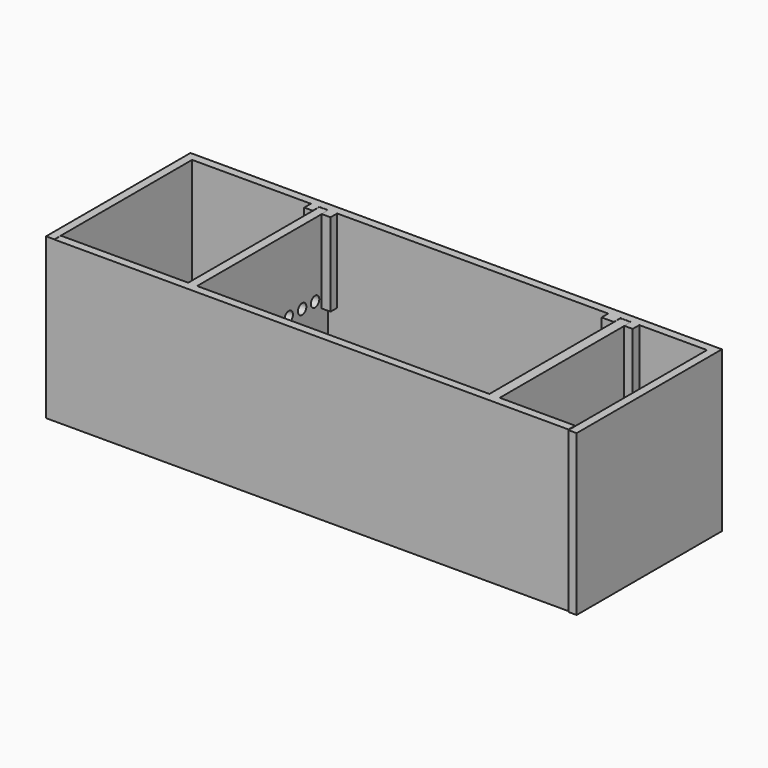
from build123d import *

# Parameters (mm, degrees)
F0_W      = 124.1378337145
F0_H      = 39.50663656
F1_DEPTH  = 3
F2_W      = 2.5017783046
F2_H      = 39.50663656
F2_W_2    = 2.1480806172
F3_DEPTH  = 17.78
F5_DEPTH  = 17.78
F7_D      = 2.54
F8_W      = 30.6726247072
F8_H      = 35.56
F8_W_2    = 18.1720815599
F8_W_3    = 70.4594738781
F9_DEPTH  = 2
F11_DEPTH = 2
F13_DEPTH = 2
F15_DEPTH = 2
F16_W     = 2.9533728957
F16_H     = 20.0437232852
F16_W_2   = 2.1480806172
F16_H_2   = 20.0032039857
F16_W_3   = 2.0457915962
F17_DEPTH = 2


with BuildPart() as f1:
    # F0 (on Top) → F1 (new body)
    with BuildSketch(Plane.XY):
        Rectangle(F0_W, F0_H)
    extrude(amount=F1_DEPTH)

    # F2 (on face) → F3 (join)
    with BuildSketch(Plane.XY.offset(3)):
        with Locations((42.4621514976, 0)):
            Rectangle(F2_W, F2_H)
        with Locations((-30.3222518414, 0)):
            Rectangle(F2_W_2, F2_H)
    extrude(amount=F3_DEPTH)

    # F5 (add): faces of the model
    f5_faces = [f1.faces().sort_by_distance(p)[0] for p in [
        (-30.3222518414, 0, 20.78),
        (42.4621514976, 0, 20.78),
    ]]
    extrude(f5_faces, amount=F5_DEPTH)

    # F7 (through all)
    with Locations(Plane(origin=(-31.39629215, 0, 0), x_dir=(0, -1, 0), z_dir=(-1, 0, 0))):
        with Locations((-11.8883280084, 20.8021104336), (-15.7889463007, 20.7917392254), (-7.8511117026, 20.7805093378), (-3.6703720689, 20.7868441939)):
            Hole(F7_D / 2)

    # F8 (on face) → F9 (join)
    with BuildSketch(Plane.XZ.offset(19.75331828)):
        Polygon((-62.0689168572, 3), (-62.0689168572, 0), (61.8851222098, 0), (61.8851222098, 3), (43.7130406499, 3), (43.7130406499, 38.56), (41.2112623453, 38.56), (41.2112623453, 3), (-29.2482115328, 3), (-29.2482115328, 38.56), (-31.39629215, 38.56), (-31.39629215, 3), align=None)
        with Locations((-46.7326045036, 20.78)):
            Rectangle(F8_W, F8_H)
        with Locations((52.7990814298, 20.78)):
            Rectangle(F8_W_2, F8_H)
        with Locations((5.9815254062, 20.78)):
            Rectangle(F8_W_3, F8_H)
    extrude(amount=F9_DEPTH)

    # F10 (on face) → F11 (join)
    with BuildSketch(Plane(origin=(0, 19.75331828, 0), x_dir=(-1, 0, 0), z_dir=(0, 1, 0))):
        Polygon((-62.0689168572, 38.6005192995), (-62.0689168572, 3), (-43.7130406499, 3), (-43.7130406499, 38.56), (-41.2112623453, 38.56), (-41.2112623453, 3), (29.2482115328, 3), (29.2482115328, 38.56), (31.39629215, 38.56), (31.39629215, 3), (62.0689168572, 3), (62.0689168572, 38.6005192995), align=None)
        Polygon((-62.0689168572, 3), (-62.0689168572, 0), (62.0689168572, 0), (62.0689168572, 3), (31.39629215, 3), (31.39629215, 38.56), (29.2482115328, 38.56), (29.2482115328, 3), (-41.2112623453, 3), (-41.2112623453, 38.56), (-43.7130406499, 38.56), (-43.7130406499, 3), align=None)
    extrude(amount=F11_DEPTH)

    # F12 (on face) → F13 (join)
    with BuildSketch(Plane.YZ.offset(62.0689168572)):
        Polygon((19.75331828, 3), (19.75331828, 38.6005192995), (-22.0371708274, 38.6005192995), (-22.0371708274, 0), (-19.75331828, 0), (-19.75331828, 3), align=None)
        Polygon((21.75331828, 0), (21.75331828, 38.6005192995), (19.75331828, 38.6005192995), (19.75331828, 3), (-19.75331828, 3), (-19.75331828, 0), align=None)
    extrude(amount=F13_DEPTH)

    # F14 (on face) → F15 (join)
    with BuildSketch(Plane(origin=(-62.0689168572, 0, 0), x_dir=(0, -1, 0), z_dir=(-1, 0, 0))):
        Polygon((-21.75331828, 0), (21.75331828, 0), (21.75331828, 38.56), (19.75331828, 38.56), (19.75331828, 3), (-19.75331828, 3), (-19.75331828, 38.6005192995), (-21.75331828, 38.6005192995), align=None)
        Polygon((19.75331828, 38.56), (21.75331828, 38.56), (21.75331828, 38.6005192995), (-19.75331828, 38.6005192995), (-19.75331828, 3), (19.75331828, 3), align=None)
    extrude(amount=F15_DEPTH)

    # F16 (on face) → F17 (join)
    with BuildSketch(Plane.XZ.offset(-19.75331828)):
        with Locations((39.7345758975, 28.5786576569)):
            Rectangle(F16_W, F16_H)
        with Locations((-30.3222518414, 28.5583980072)):
            Rectangle(F16_W_2, F16_H_2)
        Polygon((-33.4356613457, 18.5567960143), (-31.39629215, 18.5567960143), (-31.39629215, 38.56), (-31.39629215, 38.6005192995), (-33.4356613457, 38.6005192995), align=None)
        Polygon((-29.2482115328, 38.56), (-29.2482115328, 18.5567960143), (-27.0928554237, 18.5567960143), (-27.0928554237, 38.6005192995), (-29.2482115328, 38.6005192995), align=None)
        with Locations((44.735936448, 28.5786576569)):
            Rectangle(F16_W_3, F16_H)
    extrude(amount=F17_DEPTH)


solid = f1.part
